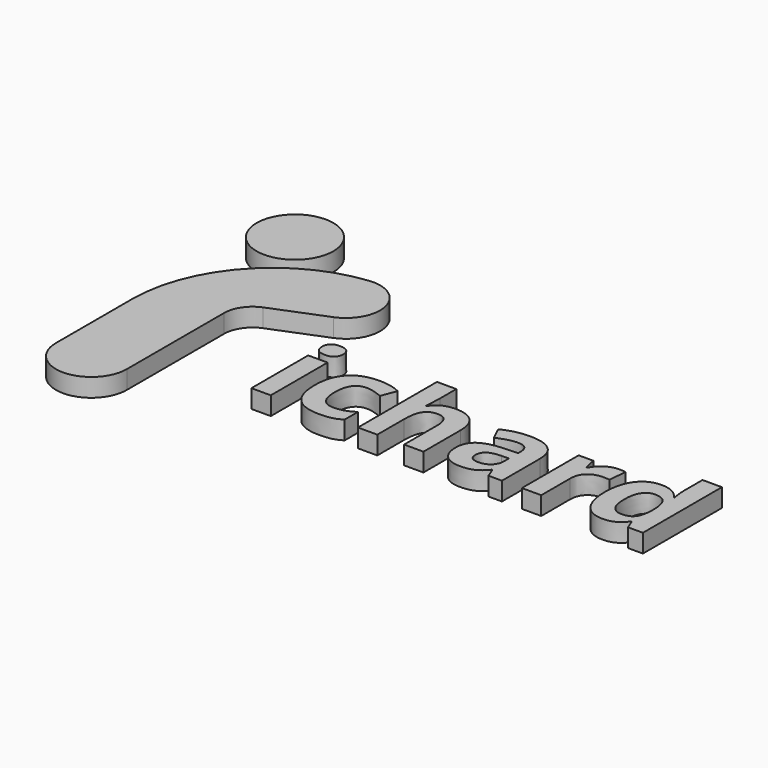
from build123d import *

# Parameters (mm, degrees)
F0_R         = 4.1831688169
F0_TEXT_SIZE = 14.1813988901
F1_DEPTH     = 2


# Not quite as in the source:
# - Text() gives the source's letters only with a copy of the font that has no kerning and outlines rounded to 1/6400 em; it was checked with that copy


with BuildPart() as f1:
    # F0 (on Top) → F1 (new body)
    with BuildSketch(Plane.XY):
        with BuildLine():
            Line((1.2644261162, 12.4899188848), (1.2644261162, 2.0905670072))
            ThreePointArc((1.2644261162, 2.0905670072), (5.1274184169, -1.7724252935), (8.9904107176, 2.0905670072))
            Line((8.9904107176, 2.0905670072), (8.9904107176, 15.3597232248))
            ThreePointArc((8.9904107176, 15.3597232248), (9.5228270994, 17.0988683519), (10.9375873197, 18.2419110002))
            Line((10.9375873197, 18.2419110002), (16.742553067, 20.5772440565))
            ThreePointArc((16.742553067, 20.5772440565), (18.9637118338, 24.9298567313), (14.9577250486, 27.7282229047))
            ThreePointArc((14.9577250486, 27.7282229047), (5.1906898007, 22.7333600187), (1.2644261162, 12.4899188848))
        make_face()
        with Locations((4.9577087204, 30.0710760518)):
            Circle(F0_R)
        with Locations((18.3650541159, 5.9868470295)):
            Text('ichard', F0_TEXT_SIZE, font='Open Sans', font_style=FontStyle.BOLD, text_align=(TextAlign.LEFT, TextAlign.BOTTOM))
    extrude(amount=F1_DEPTH)


solid = f1.part
